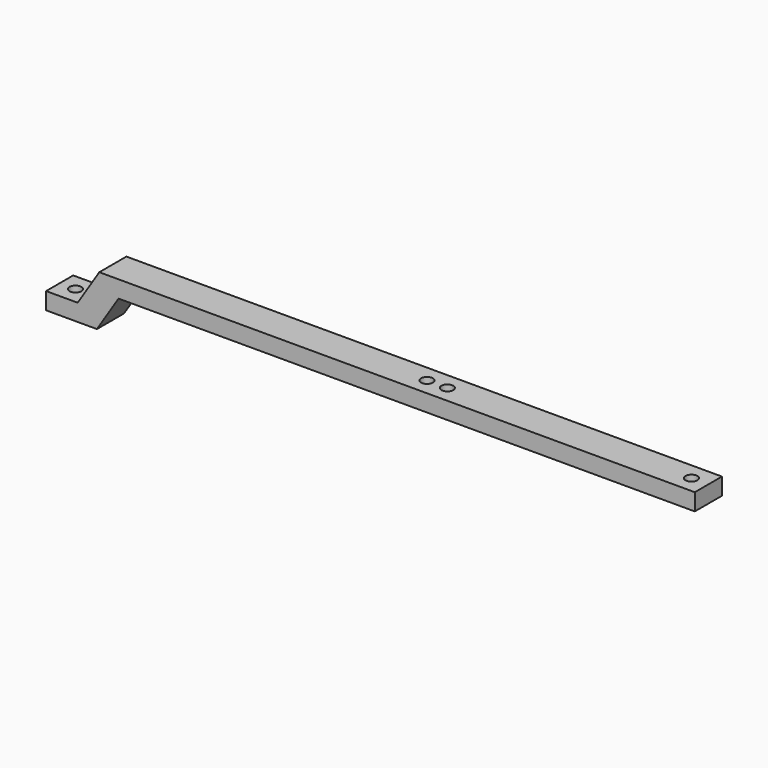
from build123d import *

# Parameters (mm, degrees)
F1_DEPTH = 10
F2_R     = 1.75
F3_DEPTH = 15.001
F5_DEPTH = 5.001


# Not quite as in the source:
# - a feature names something its author has since deleted; it is built from what else it names


with BuildPart() as f1:
    # F0 (on Front) → F1 (new body)
    with BuildSketch(Plane.XZ):
        Polygon((31.7108153552, 10), (201.7108153552, 10), (201.7108153552, 15), (30.3418431431, 15), (26.0328800881, 15), (19.6614095846, 5), (10.3393448517, 5), (10.3393448517, 0), (25.3393448517, 0), align=None)
    extrude(amount=F1_DEPTH)

    # F2 (on face) → F3 (cut, through all)
    with BuildSketch(Plane.XY.offset(15)):
        with Locations((118.7108153552, -5)):
            Circle(F2_R)
        with Locations((124.7108153552, -5)):
            Circle(F2_R)
        with Locations((196.7108153552, -5)):
            Circle(F2_R)
    extrude(amount=-F3_DEPTH, mode=Mode.SUBTRACT)

    # F4 (on face) → F5 (cut, through all)
    with BuildSketch(Plane.XY.offset(5)):
        with BuildLine():
            ThreePointArc((13.2503772181, -5), (15.0003772181, -6.75), (16.7503772181, -5))
            ThreePointArc((16.7503772181, -5), (15.0003772181, -3.25), (13.2503772181, -5))
        make_face()
    extrude(amount=-F5_DEPTH, mode=Mode.SUBTRACT)


solid = f1.part
